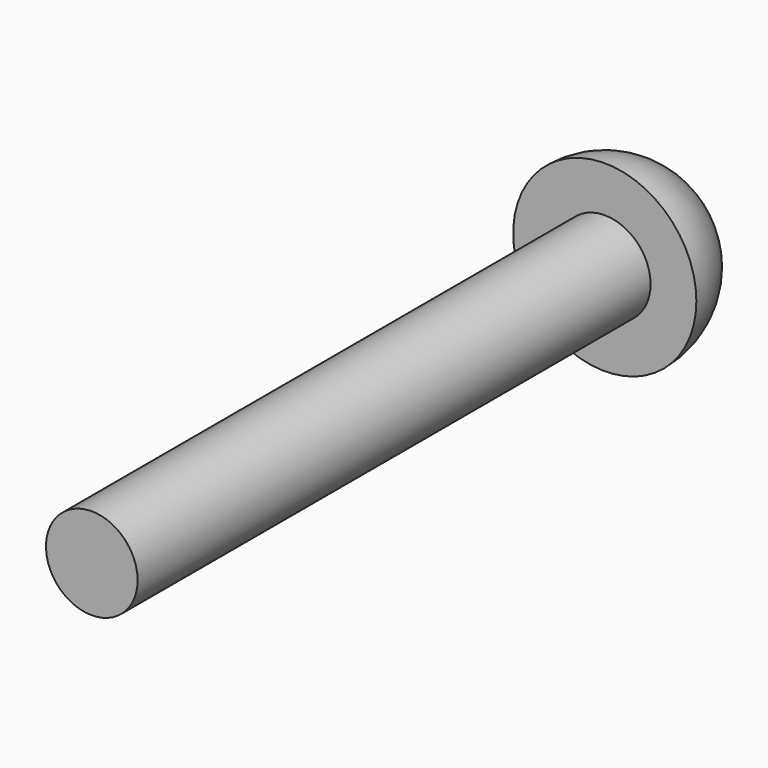
from build123d import *

# Parameters (mm, degrees)
F0_R     = 6.35
F1_DEPTH = 101.6
F2_R     = 12.7
F3_DEPTH = 12.7
F4_R     = 12.69999


# Not quite as in the source:
# - a fillet or chamfer is up to 0.001 mm smaller than in the source, because OpenCascade refuses the exact size


with BuildPart() as f1:
    # F0 (on Front) → F1 (new body)
    with BuildSketch(Plane.XZ):
        Circle(F0_R)
    extrude(amount=F1_DEPTH)

    # F2 (on Front) → F3 (join)
    with BuildSketch(Plane.XZ):
        Circle(F2_R)
    extrude(amount=F3_DEPTH)

    # F4 (radius 12.7 in the source; OpenCascade refuses exactly that, so slightly less here)
    f4_edges = [f1.edges().sort_by_distance(p)[0] for p in [
        (-12.7, 0, 0),
    ]]
    fillet(f4_edges, radius=F4_R)


solid = f1.part
